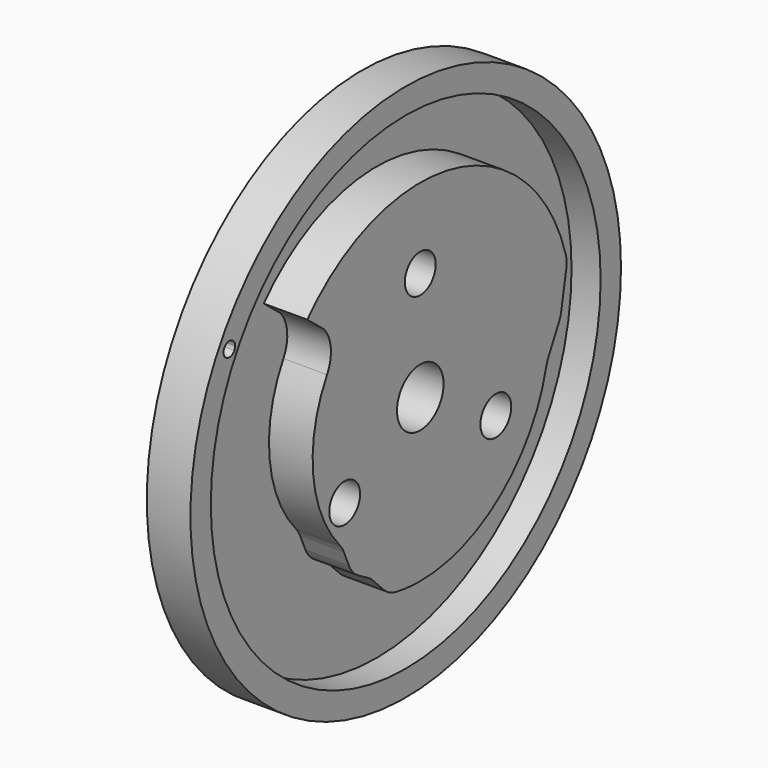
from build123d import *

# Parameters (mm, degrees)
F0_R     = 37
F0_R_2   = 2.65
F0_R_3   = 4
F1_DEPTH = 8
F2_DEPTH = 2
F3_R     = 33.5
F4_DEPTH = 4


# Not quite as in the source:
# - a feature names something its author has since deleted; it is built from what else it names


with BuildPart() as f1:
    # F0 (on Right) → F1 (new body)
    with BuildSketch(Plane.YZ):
        Circle(F0_R)
        with BuildLine():
            ThreePointArc((-31.1769145362, 18), (-30.0520700874, 18.4659258263), (-29.3108891325, 17.5))
            ThreePointArc((-29.3108891325, 17.5), (-29.3449633062, 17.2411809549), (-29.4448637287, 17))
            ThreePointArc((-29.4448637287, 17), (-30.8108891325, 16.6339745962), (-31.1769145362, 18))
        make_face(mode=Mode.SUBTRACT)
        with BuildLine():
            ThreePointArc((-13.8307570654, -12.2865845131), (-18.4050260219, -1.8721690986), (-16.02146997, 9.25))
            ThreePointArc((-16.02146997, 9.25), (-15.3688742415, 12.1652999186), (-16.4950815942, 14.9323401783))
            Line((-16.4950815942, 14.9323401783), (-19.414607735, 17.2937273743))
            ThreePointArc((-19.414607735, 17.2937273743), (5.7943493018, 25.3461144195), (25.0003908736, 7.1400599553))
            ThreePointArc((25.0003908736, 7.1400599553), (25.1492760253, 6.2395359628), (25.0901387998, 5.3287050027))
            Line((25.0901387998, 5.3287050027), (24.230588756, 0.582974524))
            ThreePointArc((24.230588756, 0.582974524), (24.0836635039, 0.0139846058), (23.8549574473, -0.527337938))
            Line((23.8549574473, -0.527337938), (22.0020362781, -4.1457144451))
            ThreePointArc((22.0020362781, -4.1457144451), (21.8067059734, -4.5923170456), (21.6671490665, -5.0593627397))
            ThreePointArc((21.6671490665, -5.0593627397), (13.8291662627, -17.4303373599), (0, -22.25))
            ThreePointArc((0, -22.25), (-2.1048516517, -22.1502166925), (-4.1908242867, -21.851761755))
            ThreePointArc((-4.1908242867, -21.851761755), (-5.3214186468, -21.4518874672), (-6.2826715748, -20.7348547893))
            Line((-6.2826715748, -20.7348547893), (-8.1615589997, -18.8334098464))
            ThreePointArc((-8.1615589997, -18.8334098464), (-8.5623101549, -18.4787752012), (-9.0068129011, -18.1808078731))
            Line((-9.0068129011, -18.1808078731), (-10.5765097016, -17.2745430028))
            ThreePointArc((-10.5765097016, -17.2745430028), (-11.5533785454, -16.4821921034), (-12.2358922377, -15.4256563749))
            Line((-12.2358922377, -15.4256563749), (-13.1618084894, -13.3279283396))
            ThreePointArc((-13.1618084894, -13.3279283396), (-13.4557617662, -12.781226145), (-13.8307570654, -12.2865845131))
        make_face(mode=Mode.SUBTRACT)
        with BuildLine():
            ThreePointArc((-16.4950815942, 14.9323401783), (-15.3688742415, 12.1652999186), (-16.02146997, 9.25))
            ThreePointArc((-16.02146997, 9.25), (-18.4050260219, -1.8721690986), (-13.8307570654, -12.2865845131))
            ThreePointArc((-13.8307570654, -12.2865845131), (-13.4557617662, -12.781226145), (-13.1618084894, -13.3279283396))
            Line((-13.1618084894, -13.3279283396), (-12.2358922377, -15.4256563749))
            ThreePointArc((-12.2358922377, -15.4256563749), (-11.5533785454, -16.4821921034), (-10.5765097016, -17.2745430028))
            Line((-10.5765097016, -17.2745430028), (-9.0068129011, -18.1808078731))
            ThreePointArc((-9.0068129011, -18.1808078731), (-8.5623101549, -18.4787752012), (-8.1615589997, -18.8334098464))
            Line((-8.1615589997, -18.8334098464), (-6.2826715748, -20.7348547893))
            ThreePointArc((-6.2826715748, -20.7348547893), (-5.3214186468, -21.4518874672), (-4.1908242867, -21.851761755))
            ThreePointArc((-4.1908242867, -21.851761755), (-2.1048516517, -22.1502166925), (0, -22.25))
            ThreePointArc((0, -22.25), (13.8291662627, -17.4303373599), (21.6671490665, -5.0593627397))
            ThreePointArc((21.6671490665, -5.0593627397), (21.8067059734, -4.5923170456), (22.0020362781, -4.1457144451))
            Line((22.0020362781, -4.1457144451), (23.8549574473, -0.527337938))
            ThreePointArc((23.8549574473, -0.527337938), (24.0836635039, 0.0139846058), (24.230588756, 0.582974524))
            Line((24.230588756, 0.582974524), (25.0901387998, 5.3287050027))
            ThreePointArc((25.0901387998, 5.3287050027), (25.1492760253, 6.2395359628), (25.0003908736, 7.1400599553))
            ThreePointArc((25.0003908736, 7.1400599553), (5.7943493018, 25.3461144195), (-19.414607735, 17.2937273743))
            Line((-19.414607735, 17.2937273743), (-16.4950815942, 14.9323401783))
        make_face()
        with Locations((-12.9903810568, -7.5)):
            Circle(F0_R_2, mode=Mode.SUBTRACT)
        with Locations((12.9903810568, -7.5)):
            Circle(F0_R_2, mode=Mode.SUBTRACT)
        Circle(F0_R_3, mode=Mode.SUBTRACT)
        with Locations((0, 15)):
            Circle(F0_R_2, mode=Mode.SUBTRACT)
    extrude(amount=-F1_DEPTH)

    # F0 (on Right) → F2 (cut)
    with BuildSketch(Plane.YZ):
        Circle(F0_R)
        with BuildLine():
            ThreePointArc((-31.1769145362, 18), (-30.0520700874, 18.4659258263), (-29.3108891325, 17.5))
            ThreePointArc((-29.3108891325, 17.5), (-29.3449633062, 17.2411809549), (-29.4448637287, 17))
            ThreePointArc((-29.4448637287, 17), (-30.8108891325, 16.6339745962), (-31.1769145362, 18))
        make_face(mode=Mode.SUBTRACT)
        with BuildLine():
            ThreePointArc((-13.8307570654, -12.2865845131), (-18.4050260219, -1.8721690986), (-16.02146997, 9.25))
            ThreePointArc((-16.02146997, 9.25), (-15.3688742415, 12.1652999186), (-16.4950815942, 14.9323401783))
            Line((-16.4950815942, 14.9323401783), (-19.414607735, 17.2937273743))
            ThreePointArc((-19.414607735, 17.2937273743), (5.7943493018, 25.3461144195), (25.0003908736, 7.1400599553))
            ThreePointArc((25.0003908736, 7.1400599553), (25.1492760253, 6.2395359628), (25.0901387998, 5.3287050027))
            Line((25.0901387998, 5.3287050027), (24.230588756, 0.582974524))
            ThreePointArc((24.230588756, 0.582974524), (24.0836635039, 0.0139846058), (23.8549574473, -0.527337938))
            Line((23.8549574473, -0.527337938), (22.0020362781, -4.1457144451))
            ThreePointArc((22.0020362781, -4.1457144451), (21.8067059734, -4.5923170456), (21.6671490665, -5.0593627397))
            ThreePointArc((21.6671490665, -5.0593627397), (13.8291662627, -17.4303373599), (0, -22.25))
            ThreePointArc((0, -22.25), (-2.1048516517, -22.1502166925), (-4.1908242867, -21.851761755))
            ThreePointArc((-4.1908242867, -21.851761755), (-5.3214186468, -21.4518874672), (-6.2826715748, -20.7348547893))
            Line((-6.2826715748, -20.7348547893), (-8.1615589997, -18.8334098464))
            ThreePointArc((-8.1615589997, -18.8334098464), (-8.5623101549, -18.4787752012), (-9.0068129011, -18.1808078731))
            Line((-9.0068129011, -18.1808078731), (-10.5765097016, -17.2745430028))
            ThreePointArc((-10.5765097016, -17.2745430028), (-11.5533785454, -16.4821921034), (-12.2358922377, -15.4256563749))
            Line((-12.2358922377, -15.4256563749), (-13.1618084894, -13.3279283396))
            ThreePointArc((-13.1618084894, -13.3279283396), (-13.4557617662, -12.781226145), (-13.8307570654, -12.2865845131))
        make_face(mode=Mode.SUBTRACT)
    extrude(amount=-F2_DEPTH, mode=Mode.SUBTRACT)

    # F3 (on face) → F4 (cut)
    with BuildSketch(Plane.YZ.offset(-2)):
        Circle(F3_R)
        with BuildLine():
            ThreePointArc((-13.8307570654, -12.2865845131), (-18.4050260219, -1.8721690986), (-16.02146997, 9.25))
            ThreePointArc((-16.02146997, 9.25), (-15.3688742415, 12.1652999186), (-16.4950815942, 14.9323401783))
            Line((-16.4950815942, 14.9323401783), (-19.414607735, 17.2937273743))
            ThreePointArc((-19.414607735, 17.2937273743), (5.7943493018, 25.3461144195), (25.0003908736, 7.1400599553))
            ThreePointArc((25.0003908736, 7.1400599553), (25.1492760253, 6.2395359628), (25.0901387998, 5.3287050027))
            Line((25.0901387998, 5.3287050027), (24.230588756, 0.582974524))
            ThreePointArc((24.230588756, 0.582974524), (24.0836635039, 0.0139846058), (23.8549574473, -0.527337938))
            Line((23.8549574473, -0.527337938), (22.0020362781, -4.1457144451))
            ThreePointArc((22.0020362781, -4.1457144451), (21.8067059734, -4.5923170456), (21.6671490665, -5.0593627397))
            ThreePointArc((21.6671490665, -5.0593627397), (12.1182361804, -18.6604086739), (-4.1908242867, -21.851761755))
            ThreePointArc((-4.1908242867, -21.851761755), (-5.3214186468, -21.4518874672), (-6.2826715748, -20.7348547893))
            Line((-6.2826715748, -20.7348547893), (-8.1615589997, -18.8334098464))
            ThreePointArc((-8.1615589997, -18.8334098464), (-8.5623101549, -18.4787752012), (-9.0068129011, -18.1808078731))
            Line((-9.0068129011, -18.1808078731), (-10.5765097016, -17.2745430028))
            ThreePointArc((-10.5765097016, -17.2745430028), (-11.5533785454, -16.4821921034), (-12.2358922377, -15.4256563749))
            Line((-12.2358922377, -15.4256563749), (-13.1618084894, -13.3279283396))
            ThreePointArc((-13.1618084894, -13.3279283396), (-13.4557617662, -12.781226145), (-13.8307570654, -12.2865845131))
        make_face(mode=Mode.SUBTRACT)
    extrude(amount=-F4_DEPTH, mode=Mode.SUBTRACT)


solid = f1.part
